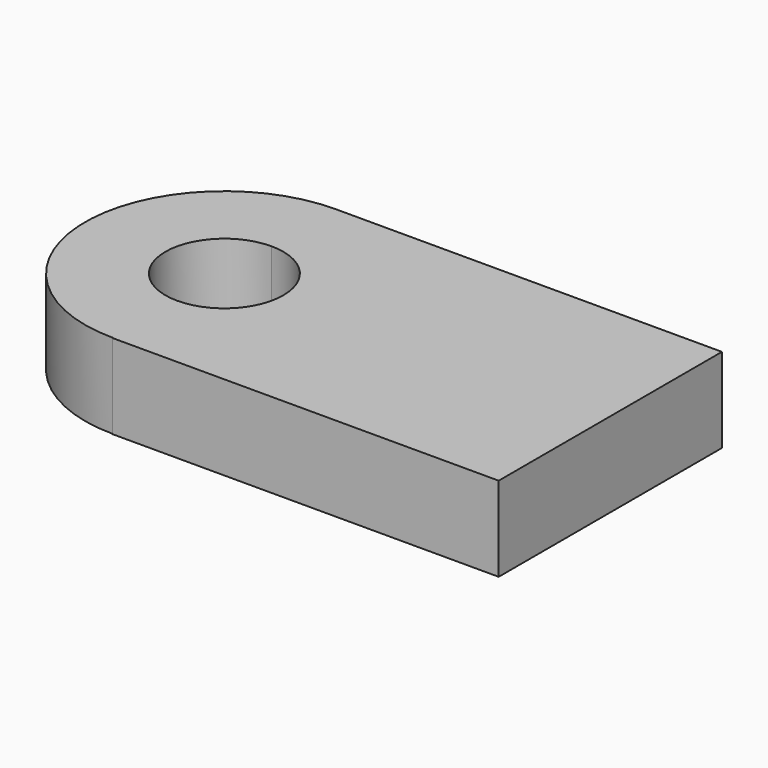
from build123d import *
from build123d import SkipClean  # not in build123d's __all__

# Parameters (mm, degrees)
F1_DEPTH  = 25.4
F1_FACE_R = 17.6985452631
F2_DEPTH  = 25.4
F3_DEPTH  = 25.4


with BuildPart() as f1:
    # F0 (on Top) → F1 (new body)
    with BuildSketch(Plane.XY):
        with BuildLine():
            ThreePointArc((0, 41.7947099158), (29.5533227992, 29.5533227992), (41.7947099158, 0))
            ThreePointArc((41.7947099158, 0), (29.5533227992, -29.5533227992), (0, -41.7947099158))
            Line((0, -41.7947099158), (0, -41.9407263398))
            Line((0, -41.9407263398), (115.8670112491, -41.9407263398))
            Line((115.8670112491, -41.9407263398), (115.8670112491, 41.7947099158))
            Line((115.8670112491, 41.7947099158), (0, 41.7947099158))
        make_face()
        with BuildLine():
            ThreePointArc((0, -41.7947099158), (29.5533227992, -29.5533227992), (41.7947099158, 0))
            ThreePointArc((41.7947099158, 0), (29.5533227992, 29.5533227992), (0, 41.7947099158))
            Line((0, 41.7947099158), (0, 17.6985452631))
            ThreePointArc((0, 17.6985452631), (12.5147613727, 12.5147613727), (17.6985452631, 0))
            ThreePointArc((17.6985452631, 0), (12.5147613727, -12.5147613727), (0, -17.6985452631))
            Line((0, -17.6985452631), (0, -41.7947099158))
        make_face()
        with BuildLine():
            Line((0, 17.6985452631), (0, 41.7947099158))
            ThreePointArc((0, 41.7947099158), (-41.7947099158, 0), (0, -41.7947099158))
            Line((0, -41.7947099158), (0, -17.6985452631))
            ThreePointArc((0, -17.6985452631), (-17.6985452631, 0), (0, 17.6985452631))
        make_face()
    extrude(amount=F1_DEPTH)

    # F1_face (on face) + F0 (on Top) → F2 (join)
    with BuildSketch(Plane(origin=(44.792448598, -0.0617990101, 25.4), x_dir=(1, 0, 0), z_dir=(0, 0, 1))):
        with BuildLine():
            Line((71.0745626511, 41.8565089259), (-44.792448598, 41.8565089259))
            ThreePointArc((-44.792448598, 41.8565089259), (-86.5871585138, 0.0617990101), (-44.792448598, -41.7329109057))
            Line((-44.792448598, -41.7329109057), (-44.792448598, -41.8789273297))
            Line((-44.792448598, -41.8789273297), (71.0745626511, -41.8789273297))
            Line((71.0745626511, -41.8789273297), (71.0745626511, 41.8565089259))
        make_face()
        with Locations((-44.792448598, 0.0617990101)):
            Circle(F1_FACE_R, mode=Mode.SUBTRACT)
    with BuildSketch(Plane.XY):
        with BuildLine():
            ThreePointArc((0, -41.7947099158), (29.5533227992, -29.5533227992), (41.7947099158, 0))
            ThreePointArc((41.7947099158, 0), (29.5533227992, 29.5533227992), (0, 41.7947099158))
            Line((0, 41.7947099158), (0, 17.6985452631))
            ThreePointArc((0, 17.6985452631), (12.5147613727, 12.5147613727), (17.6985452631, 0))
            ThreePointArc((17.6985452631, 0), (12.5147613727, -12.5147613727), (0, -17.6985452631))
            Line((0, -17.6985452631), (0, -41.7947099158))
        make_face()
        with BuildLine():
            ThreePointArc((0, 41.7947099158), (29.5533227992, 29.5533227992), (41.7947099158, 0))
            ThreePointArc((41.7947099158, 0), (29.5533227992, -29.5533227992), (0, -41.7947099158))
            Line((0, -41.7947099158), (0, -41.9407263398))
            Line((0, -41.9407263398), (115.8670112491, -41.9407263398))
            Line((115.8670112491, -41.9407263398), (115.8670112491, 41.7947099158))
            Line((115.8670112491, 41.7947099158), (0, 41.7947099158))
        make_face()
        with BuildLine():
            Line((0, 17.6985452631), (0, 41.7947099158))
            ThreePointArc((0, 41.7947099158), (-41.7947099158, 0), (0, -41.7947099158))
            Line((0, -41.7947099158), (0, -17.6985452631))
            ThreePointArc((0, -17.6985452631), (-17.6985452631, 0), (0, 17.6985452631))
        make_face()
    with SkipClean():  # cleaning this boolean's faces spoils the solid; the shape is the same uncleaned
        extrude(amount=F2_DEPTH)

    # F3 (cut): a face of the model
    f3_faces = [f1.faces().sort_by_distance(p)[0] for p in [
        (44.792448598, -0.0617990101, 50.8),
    ]]
    extrude(f3_faces, amount=-F3_DEPTH, mode=Mode.SUBTRACT)


solid = f1.part
